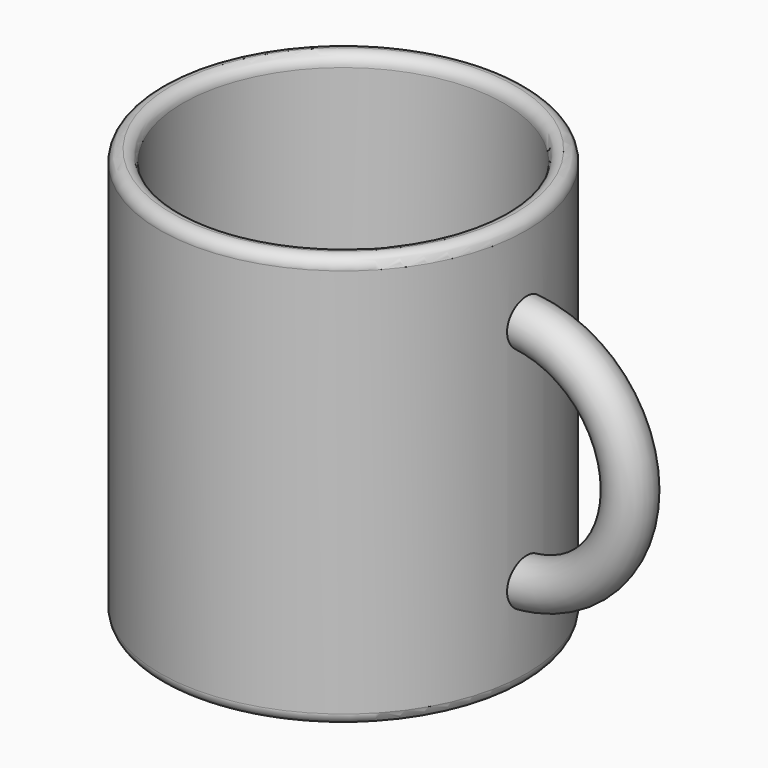
from build123d import *

# Parameters (mm, degrees)
F0_R     = 40
F1_DEPTH = 90
F2_T     = -5
F4_R     = 5
F5_ANGLE = 180
F6_R     = 2.49999
F7_R     = 2.5


# Not quite as in the source:
# - a fillet or chamfer is up to 0.001 mm smaller than in the source, because OpenCascade refuses the exact size


with BuildPart() as f1:
    # F0 (on Top) → F1 (new body)
    with BuildSketch(Plane.XY):
        Circle(F0_R)
    extrude(amount=F1_DEPTH)

    # F2
    f2_openings = [f1.faces().sort_by_distance(p)[0] for p in [
        (0, 0, 90),
    ]]
    offset(amount=F2_T, openings=f2_openings)

    # F4 (on offset) → F5 (revolve)
    with BuildSketch(Plane.YZ.offset(37.5)):
        with Locations((0, 70)):
            Circle(F4_R)
    revolve(axis=Axis((37.5, 33.2942344248, 45), (0, 1, 0)), revolution_arc=F5_ANGLE)

    # F6 (radius 2.5 in the source; OpenCascade refuses exactly that, so slightly less here)
    f6_edges = [f1.edges().sort_by_distance(p)[0] for p in [
        (-40, 0, 90),
        (-35, 0, 90),
    ]]
    fillet(f6_edges, radius=F6_R)

    # F7
    f7_edges = [f1.edges().sort_by_distance(p)[0] for p in [
        (-40, 0, 0),
    ]]
    fillet(f7_edges, radius=F7_R)


solid = f1.part
